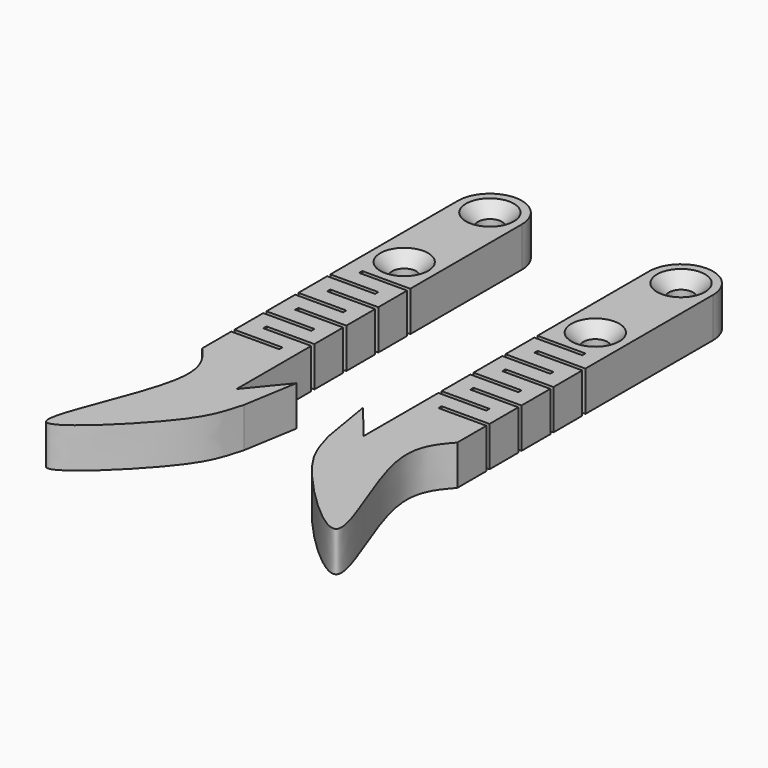
from build123d import *

# Parameters (mm, degrees)
F0_R     = 1.905
F1_DEPTH = 6.35
F2_SIZE  = 1.905


# Not quite as in the source:
# - a feature names something its author has since deleted; it is built from what else it names


with BuildPart() as f1:
    # F0 (on Top) → F1 (new body)
    with BuildSketch(Plane.XY):
        with BuildLine():
            Line((0.635, 32.3274787827), (-2.54, 32.3274787827))
            ThreePointArc((-2.54, 32.3274787827), (2.54, 27.2474787827), (7.62, 32.3274787827))
            Line((7.62, 32.3274787827), (4.445, 32.3274787827))
            ThreePointArc((4.445, 32.3274787827), (2.54, 30.4224787827), (0.635, 32.3274787827))
        make_face()
        with BuildLine():
            ThreePointArc((7.62, 32.3274787827), (2.54, 37.4074787827), (-2.54, 32.3274787827))
            Line((-2.54, 32.3274787827), (0.635, 32.3274787827))
            ThreePointArc((0.635, 32.3274787827), (2.54, 34.2324787827), (4.445, 32.3274787827))
            Line((4.445, 32.3274787827), (7.62, 32.3274787827))
        make_face()
        with BuildLine():
            Line((-2.54, -9.525), (-2.54, -18.4725212173))
            Line((-2.54, -18.4725212173), (-2.54, -24.3690894357))
            Line((-2.54, -24.3690894357), (-7.3664773123, -18.4725212173))
            Line((-7.3664773123, -18.4725212173), (-5.9221661487, -27.1184083573))
            add(Edge.make_bspline(
                [(-5.9221661487, -27.1184083573), (-5.0940429792, -29.8072900623), (-4.4350836246, -34.076325633), (17.6067707768, -55.5132531587), (1.6726871659, -25.297889833), (5.911566797, -20.4156751081), (7.62, -18.4725212173)],
                knots=[0, 0, 0, 0, 0.2021996559, 0.4867073763, 0.7982350217, 1, 1, 1, 1], degree=3))
            Line((7.62, -18.4725212173), (7.62, -12.7))
            Line((7.62, -12.7), (0, -12.7))
            Line((0, -12.7), (0, -12.065))
            Line((0, -12.065), (7.62, -12.065))
            Line((7.62, -12.065), (7.62, -6.35))
            Line((7.62, -6.35), (0, -6.35))
            Line((0, -6.35), (0, -5.715))
            Line((0, -5.715), (7.62, -5.715))
            Line((7.62, -5.715), (7.62, 0))
            Line((7.62, 0), (0, 0))
            Line((0, 0), (0, 0.635))
            Line((0, 0.635), (7.62, 0.635))
            Line((7.62, 0.635), (7.62, 6.35))
            Line((7.62, 6.35), (0, 6.35))
            Line((0, 6.35), (0, 6.985))
            Line((0, 6.985), (5.9817770534, 6.985))
            Line((5.9817770534, 6.985), (7.62, 6.985))
            Line((7.62, 6.985), (7.62, 9.525))
            Line((7.62, 9.525), (7.62, 32.3274787827))
            ThreePointArc((7.62, 32.3274787827), (2.54, 27.2474787827), (-2.54, 32.3274787827))
            Line((-2.54, 32.3274787827), (-2.54, 19.6274787827))
            Line((-2.54, 19.6274787827), (-2.54, 10.16))
            Line((-2.54, 10.16), (5.08, 10.16))
            Line((5.08, 10.16), (5.08, 9.525))
            Line((5.08, 9.525), (-2.54, 9.525))
            Line((-2.54, 9.525), (-2.54, 3.81))
            Line((-2.54, 3.81), (5.08, 3.81))
            Line((5.08, 3.81), (5.08, 3.175))
            Line((5.08, 3.175), (-2.54, 3.175))
            Line((-2.54, 3.175), (-2.54, -2.54))
            Line((-2.54, -2.54), (5.08, -2.54))
            Line((5.08, -2.54), (5.08, -3.175))
            Line((5.08, -3.175), (-2.54, -3.175))
            Line((-2.54, -3.175), (-2.54, -8.89))
            Line((-2.54, -8.89), (5.08, -8.89))
            Line((5.08, -8.89), (5.08, -9.525))
            Line((5.08, -9.525), (-2.54, -9.525))
        make_face()
        with Locations((2.54, 15.3047889471)):
            Circle(F0_R, mode=Mode.SUBTRACT)
    extrude(amount=F1_DEPTH)

    # F2
    f2_edges = [f1.edges().sort_by_distance(p)[0] for p in [
        (0.635, 15.304789, 6.35),
        (4.445, 32.327479, 6.35),
    ]]
    chamfer(f2_edges, length=F2_SIZE)


with BuildPart() as f5_1:
    # F5: instance of F1
    add(f1.part.mirror(Plane(origin=(-12.6467412338, 13.2919847965, 12.7), x_dir=(0, 1, 0), z_dir=(1, 0, 0))))


solid = Compound([f1.part, f5_1.part])
